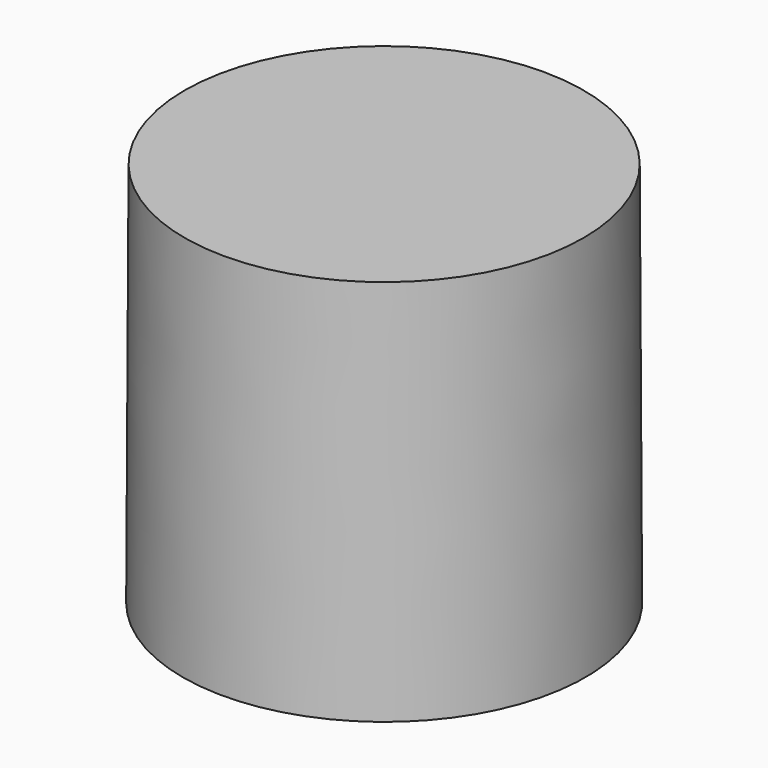
from build123d import *


with BuildPart() as f1:
    # F0 (on Front) → F1 (revolve)
    with BuildSketch(Plane.XZ):
        Polygon((-16.5608, 0), (0, 0), (0, 31.75), (-16.4084, 31.75), align=None)
    revolve(axis=Axis((0, 0, 15.875), (0, 0, 1)))

    # F2 (on Front) → F3 (revolve, cut)
    with BuildSketch(Plane.XZ):
        Polygon((-11.938, 0), (0, 0), (0, 19.558), (-11.8364, 19.558), align=None)
    revolve(axis=Axis((0, 0, 9.779), (0, 0, 1)), mode=Mode.SUBTRACT)


solid = f1.part
